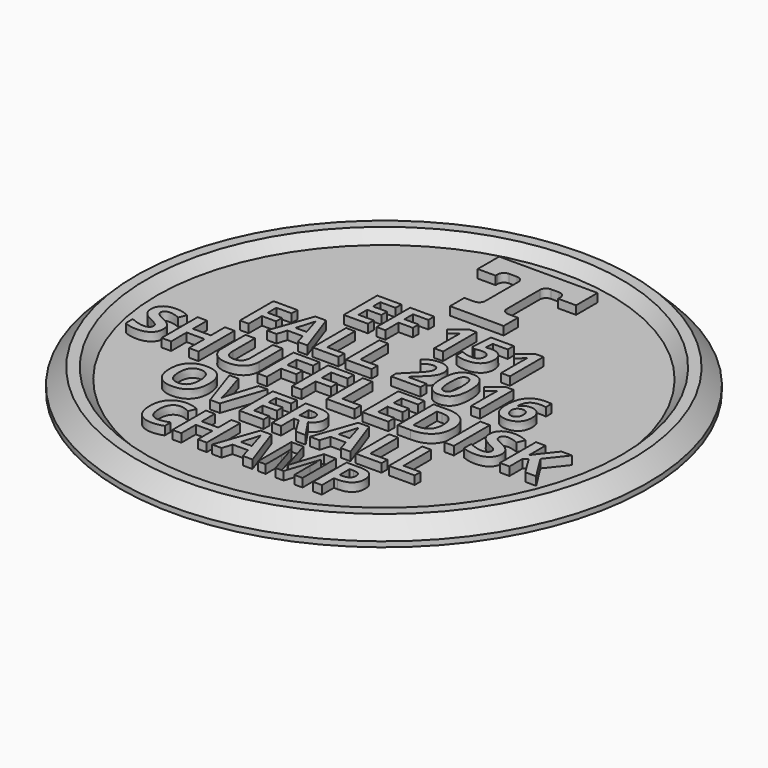
from build123d import *

# Parameters (mm, degrees)
F0_W           = 25
F0_H           = 2
F2_R           = 22.5
F3_DEPTH       = 1
F3_TAPER       = 45
F5_SIZE        = 1.5
F4_TEXT_SIZE   = 5.5555555556
F4_TEXT_SIZE_2 = 5.9722222222
F6_DEPTH       = 0.8


# Not quite as in the source:
# - Text() gives the source's letters only with a copy of the font that has no kerning and outlines rounded to 1/6400 em; it was checked with that copy


with BuildPart() as f1:
    # F0 (on Right) → F1 (revolve)
    with BuildSketch(Plane.YZ):
        with Locations((12.5, 1)):
            Rectangle(F0_W, F0_H)
    revolve(axis=Axis((0, 0, 1), (0, 0, 1)))

    # F2 (on face) → F3 (cut)
    with BuildSketch(Plane.XY.offset(2)):
        Circle(F2_R)
    extrude(amount=-F3_DEPTH, taper=F3_TAPER, mode=Mode.SUBTRACT)

    # F5
    f5_edges = [f1.edges().sort_by_distance(p)[0] for p in [
        (0, -25, 2),
    ]]
    chamfer(f5_edges, length=F5_SIZE)

    # F4 (on face) → F6 (join)
    with BuildSketch(Plane.XY.offset(1)):
        with BuildLine():
            Line((-4.6566666667, 19.4666666667), (-4.6566666667, 16.9266666667))
            Line((-4.6566666667, 16.9266666667), (-2.9633333333, 16.9266666667))
            Line((-2.9633333333, 16.9266666667), (-2.9633333333, 17.1806666667))
            ThreePointArc((-2.9633333333, 17.1806666667), (-2.7897452856, 17.5997452856), (-2.3706666667, 17.7733333333))
            Line((-2.3706666667, 17.7733333333), (-1.6086666667, 17.7733333333))
            ThreePointArc((-1.6086666667, 17.7733333333), (-1.1895880477, 17.5997452856), (-1.016, 17.1806666667))
            Line((-1.016, 17.1806666667), (-1.016, 13.286))
            ThreePointArc((-1.016, 13.286), (-1.1895880477, 12.866921381), (-1.6086666667, 12.6933333333))
            Line((-1.6086666667, 12.6933333333), (-2.54, 12.6933333333))
            Line((-2.54, 12.6933333333), (-2.54, 11))
            Line((-2.54, 11), (0, 11))
            Line((0, 11), (0, 19.4666666667))
            Line((0, 19.4666666667), (-4.6566666667, 19.4666666667))
        make_face()
        with BuildLine():
            Line((4.6566666667, 19.4666666667), (0, 19.4666666667))
            Line((0, 19.4666666667), (0, 11))
            Line((0, 11), (2.54, 11))
            Line((2.54, 11), (2.54, 12.6933333333))
            Line((2.54, 12.6933333333), (1.6086666667, 12.6933333333))
            ThreePointArc((1.6086666667, 12.6933333333), (1.1895880477, 12.866921381), (1.016, 13.286))
            Line((1.016, 13.286), (1.016, 17.1806666667))
            ThreePointArc((1.016, 17.1806666667), (1.1895880477, 17.5997452856), (1.6086666667, 17.7733333333))
            Line((1.6086666667, 17.7733333333), (2.3706666667, 17.7733333333))
            ThreePointArc((2.3706666667, 17.7733333333), (2.7897452856, 17.5997452856), (2.9633333333, 17.1806666667))
            Line((2.9633333333, 17.1806666667), (2.9633333333, 16.9266666667))
            Line((2.9633333333, 16.9266666667), (4.6566666667, 16.9266666667))
            Line((4.6566666667, 16.9266666667), (4.6566666667, 19.4666666667))
        make_face()
        with Locations((-13.7361111111, -0.5)):
            Text('FALL 2016', F4_TEXT_SIZE, font='Open Sans', font_style=FontStyle.BOLD, text_align=(TextAlign.LEFT, TextAlign.BOTTOM))
        with Locations((-19.8450412326, -6.3)):
            Text('SHUFFLEDISK', F4_TEXT_SIZE_2, font='Open Sans', font_style=FontStyle.BOLD, text_align=(TextAlign.LEFT, TextAlign.BOTTOM))
        with Locations((-10.23046875, -17.3)):
            Text('CHAMP', F4_TEXT_SIZE, font='Open Sans', font_style=FontStyle.BOLD, text_align=(TextAlign.LEFT, TextAlign.BOTTOM))
        with Locations((-8.30078125, 5)):
            Text('EF 151', F4_TEXT_SIZE, font='Open Sans', font_style=FontStyle.BOLD, text_align=(TextAlign.LEFT, TextAlign.BOTTOM))
        with Locations((-12.7855034722, -11.8)):
            Text('OVER', F4_TEXT_SIZE, font='Open Sans', font_style=FontStyle.BOLD, text_align=(TextAlign.LEFT, TextAlign.BOTTOM))
        with Locations((2.4355034722, -11.8)):
            Text('ALL', F4_TEXT_SIZE, font='Open Sans', font_style=FontStyle.BOLD, text_align=(TextAlign.LEFT, TextAlign.BOTTOM))
    extrude(amount=F6_DEPTH)


solid = f1.part
